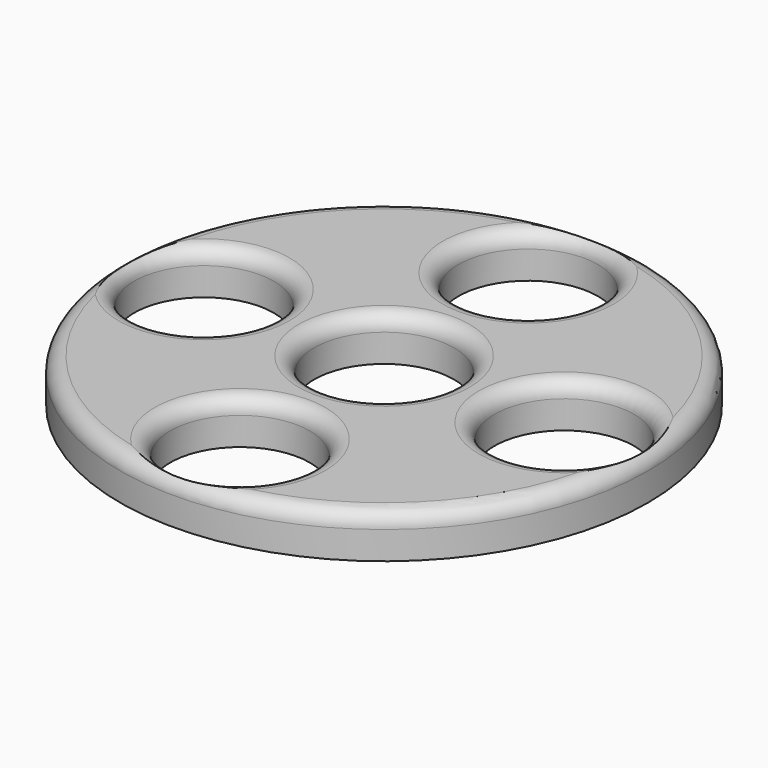
from build123d import *

# Parameters (mm, degrees)
F0_R     = 42.5
F0_R_2   = 11.25
F1_DEPTH = 7


# Not quite as in the source:
# - a fillet or chamfer that OpenCascade refuses, or shapes differently, is made with other operations: its cross-section is extruded or revolved along the edge and cut away or added


with BuildPart() as f1:
    # F0 (on Top) → F1 (new body)
    with BuildSketch(Plane.XY):
        Circle(F0_R)
        with Locations((0, -29.0052499622)):
            Circle(F0_R_2, mode=Mode.SUBTRACT)
        with Locations((-29.0052499622, 0)):
            Circle(F0_R_2, mode=Mode.SUBTRACT)
        Circle(F0_R_2, mode=Mode.SUBTRACT)
        with Locations((29.0052499622, 0)):
            Circle(F0_R_2, mode=Mode.SUBTRACT)
        with Locations((0, 29.0052499622)):
            Circle(F0_R_2, mode=Mode.SUBTRACT)
    extrude(amount=F1_DEPTH)

    # F2: fillet of radius 2.5 on 6 edges, made by hand

    # F2_s1 → F2_t2 (revolve, cut)
    with BuildSketch(Plane.XZ):
        with BuildLine():
            ThreePointArc((42.5, 4.5), (41.767766953, 6.267766953), (40, 7))
            Line((40, 7), (42.5, 7))
            Line((42.5, 7), (42.5, 4.5))
        make_face()
    revolve(axis=Axis((0, 0, 7), (0, 0, 1)), mode=Mode.SUBTRACT)

    # F2_s3 → F2_t4 (revolve, cut)
    with BuildSketch(Plane.XZ.offset(29.0052499622)):
        with BuildLine():
            ThreePointArc((11.25, 4.5), (11.982233047, 6.267766953), (13.75, 7))
            Line((13.75, 7), (11.25, 7))
            Line((11.25, 7), (11.25, 4.5))
        make_face()
    revolve(axis=Axis((0, -29.0052499622, 7), (0, 0, 1)), mode=Mode.SUBTRACT)

    # F2_s5 → F2_t6 (revolve, cut)
    with BuildSketch(Plane.XZ):
        with BuildLine():
            ThreePointArc((-17.7552499622, 4.5), (-17.0230169152, 6.267766953), (-15.2552499622, 7))
            Line((-15.2552499622, 7), (-17.7552499622, 7))
            Line((-17.7552499622, 7), (-17.7552499622, 4.5))
        make_face()
    revolve(axis=Axis((-29.0052499622, 0, 7), (0, 0, 1)), mode=Mode.SUBTRACT)

    # F2_s7 → F2_t8 (revolve, cut)
    with BuildSketch(Plane.XZ):
        with BuildLine():
            ThreePointArc((11.25, 4.5), (11.982233047, 6.267766953), (13.75, 7))
            Line((13.75, 7), (11.25, 7))
            Line((11.25, 7), (11.25, 4.5))
        make_face()
    revolve(axis=Axis((0, 0, 7), (0, 0, 1)), mode=Mode.SUBTRACT)

    # F2_s9 → F2_t10 (revolve, cut)
    with BuildSketch(Plane.XZ):
        with BuildLine():
            ThreePointArc((40.2552499622, 4.5), (40.9874830092, 6.267766953), (42.7552499622, 7))
            Line((42.7552499622, 7), (40.2552499622, 7))
            Line((40.2552499622, 7), (40.2552499622, 4.5))
        make_face()
    revolve(axis=Axis((29.0052499622, 0, 7), (0, 0, 1)), mode=Mode.SUBTRACT)

    # F2_s11 → F2_t12 (revolve, cut)
    with BuildSketch(Plane.XZ.offset(-29.0052499622)):
        with BuildLine():
            ThreePointArc((11.25, 4.5), (11.982233047, 6.267766953), (13.75, 7))
            Line((13.75, 7), (11.25, 7))
            Line((11.25, 7), (11.25, 4.5))
        make_face()
    revolve(axis=Axis((0, 29.0052499622, 7), (0, 0, 1)), mode=Mode.SUBTRACT)


solid = f1.part
